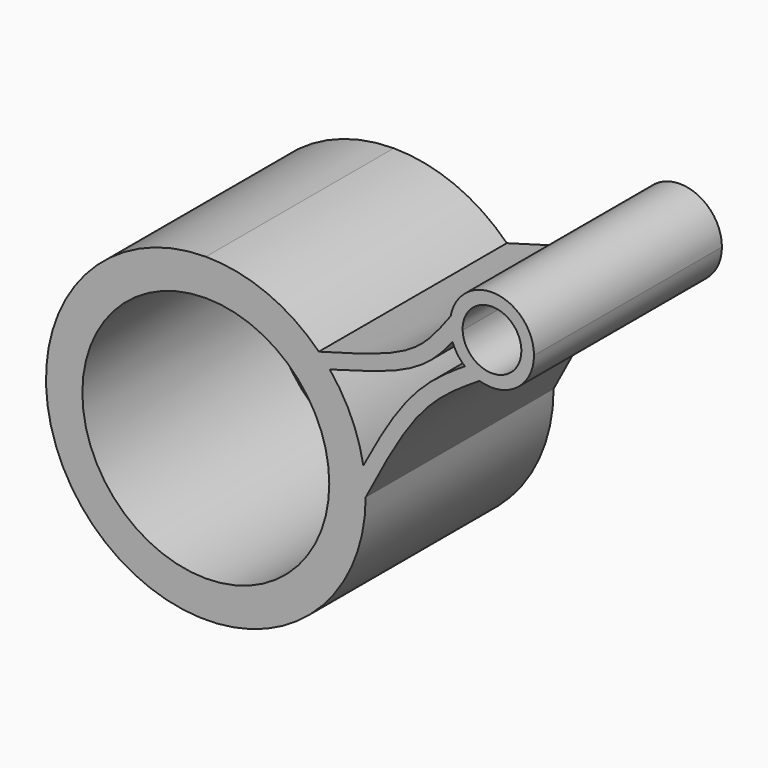
from build123d import *

# Parameters (mm, degrees)
F1_DEPTH = 40


# Not quite as in the source:
# - the dataset's text gives a spline's control points without its knots; the knots are read off the source's solid


with BuildPart() as f1:
    # F0 (on Front) → F1 (new body)
    with BuildSketch(Plane.XZ):
        with BuildLine():
            Line((14.8645307095, 14.8645307095), (19.2446576564, 19.2446576564))
            ThreePointArc((19.2446576564, 19.2446576564), (10.4151336723, 25.1443569656), (0, 27.2160558609))
            Line((0, 27.2160558609), (0, 21.0216209277))
            ThreePointArc((0, 21.0216209277), (8.0446260505, 19.4214453153), (14.8645307095, 14.8645307095))
        make_face()
        with BuildLine():
            add(Edge.make_bspline(
                [(19.2446576564, 19.2446576564), (24.6689861063, 20.8169419681), (35.6038275727, 23.3831834597), (39.5588464284, 29.0400313178), (41.6940481575, 31.8752741371)],
                knots=[0, 0, 0, 0, 0.5609906845, 0.9958506588, 0.9958506588, 0.9958506588, 0.9958506588], degree=3))
            ThreePointArc((19.2446576564, 19.2446576564), (20.2037869779, 18.2351498041), (21.1100269664, 17.1779061036))
            add(Edge.make_bspline(
                [(21.1100269664, 17.1779061036), (21.932882048, 17.4106073742), (24.0175916845, 17.9893669374), (27.419341518, 18.9554948799), (30.5229232771, 19.9727275496), (32.8770808493, 20.9067554384), (34.2794910559, 21.5551214884), (35.3497904598, 22.1226810179), (36.1267174841, 22.5777216487), (36.8651895753, 23.0595386993), (37.7916316161, 23.7289766273), (38.8502830375, 24.6135981903), (40.3593073263, 26.1032349307), (41.3483421725, 27.3012382121), (41.9852374937, 28.1182048261), (42.0071509342, 28.1463677389)],
                knots=[0.0404952119, 0.0404952119, 0.0404952119, 0.0404952119, 0.125, 0.25, 0.375, 0.4375, 0.5, 0.53125, 0.5625, 0.59375, 0.625, 0.6875, 0.75, 0.875, 0.8794611677, 0.8794611677, 0.8794611677, 0.8794611677], degree=3))
            ThreePointArc((42.0071509342, 28.1463677389), (41.602326035, 29.9899743097), (41.6940481575, 31.8752741371))
        make_face()
        with BuildLine():
            ThreePointArc((21.1100269664, 17.1779061036), (20.2037869779, 18.2351498041), (19.2446576564, 19.2446576564))
            Line((19.2446576564, 19.2446576564), (14.8645307095, 14.8645307095))
            ThreePointArc((14.8645307095, 14.8645307095), (19.4214453153, 8.0446260505), (21.0216209277, 0))
            Line((21.0216209277, 0), (27.2160558609, 0))
            ThreePointArc((27.2160558609, 0), (27.1163610427, 2.3273720003), (26.8180069698, 4.6376932618))
            ThreePointArc((26.8180069698, 4.6376932618), (24.7707154474, 11.2749879312), (21.1100269664, 17.1779061036))
        make_face()
        with BuildLine():
            Line((0, 21.0216209277), (0, 27.2160558609))
            ThreePointArc((0, 27.2160558609), (-19.2446576564, -19.2446576564), (27.2160558609, 0))
            Line((27.2160558609, 0), (21.0216209277, 0))
            ThreePointArc((21.0216209277, 0), (-14.8645307095, -14.8645307095), (0, 21.0216209277))
        make_face()
        with BuildLine():
            ThreePointArc((55.8771080393, 30.5882225912), (49.3733508957, 37.7088912623), (41.6940481575, 31.8752741371))
            ThreePointArc((41.6940481575, 31.8752741371), (41.602326035, 29.9899743097), (42.0071509342, 28.1463677389))
            ThreePointArc((42.0071509342, 28.1463677389), (42.8595475903, 26.5025969086), (44.1054687849, 25.1328367183))
            ThreePointArc((44.1054687849, 25.1328367183), (45.2874793483, 24.3200561007), (46.60794615, 23.7595842193))
            ThreePointArc((46.60794615, 23.7595842193), (52.9679994545, 24.8317552686), (55.8771080393, 30.5882225912))
        make_face()
        with BuildLine():
            ThreePointArc((53.7271809085, 30.5882225912), (48.8098673687, 25.588906343), (43.7299157288, 30.4228722856))
            ThreePointArc((43.7299157288, 30.4228722856), (48.6444944483, 35.5875388394), (53.7271809085, 30.5882225912))
        make_face(mode=Mode.SUBTRACT)
        with BuildLine():
            ThreePointArc((26.8180069698, 4.6376932618), (27.1163610427, 2.3273720003), (27.2160558609, 0))
            add(Edge.make_bspline(
                [(27.2160558609, 0), (30.4118613071, 6.1535153267), (36.1085642411, 17.1225033402), (43.4048284049, 21.734764605), (46.60794615, 23.7595842193)],
                knots=[0, 0, 0, 0, 0.5609920336, 1, 1, 1, 1], degree=3))
            ThreePointArc((46.60794615, 23.7595842193), (45.2874793483, 24.3200561007), (44.1054687849, 25.1328367183))
            add(Edge.make_bspline(
                [(26.8180069698, 4.6376932618), (26.9287178391, 4.8472219351), (27.763643844, 6.4224538826), (29.3467248011, 9.3274546207), (31.2690824478, 12.5225076847), (32.8847011617, 14.9107917128), (33.9343354718, 16.3212905579), (34.8023613487, 17.3919432452), (35.693376161, 18.4237208714), (36.8375292868, 19.6172523124), (38.236939936, 20.9022131544), (40.1258580525, 22.4490696098), (42.0976326485, 23.8377548069), (43.5711967417, 24.7916786126), (44.1054687849, 25.1328367183)],
                knots=[0.1058501262, 0.1058501262, 0.1058501262, 0.1058501262, 0.125, 0.25, 0.375, 0.4375, 0.5, 0.53125, 0.5625, 0.625, 0.6875, 0.75, 0.875, 0.9471213486, 0.9471213486, 0.9471213486, 0.9471213486], degree=3))
        make_face()
    extrude(amount=F1_DEPTH)


solid = f1.part
